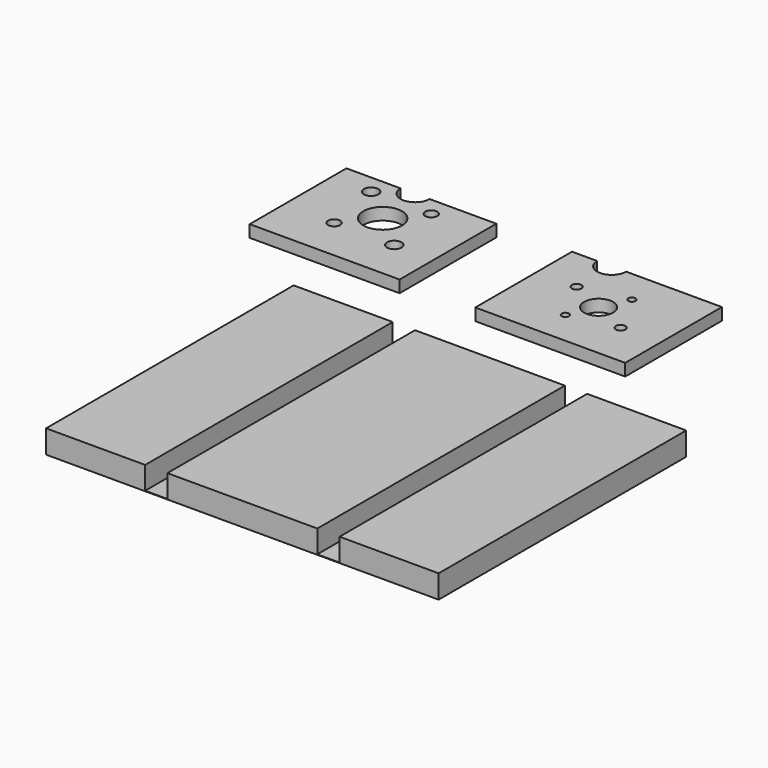
from build123d import *

# Parameters (mm, degrees)
F1_R     = 0.75
F1_R_2   = 1
F1_R_3   = 3
F4_DEPTH = 2.5
F2_R     = 1.25
F2_R_2   = 1.5
F2_R_3   = 4
F3_W     = 4.6
F3_H     = 64
F5_DEPTH = 0.1
F6_DEPTH = 4.7


# Not quite as in the source:
# - ends of sketch curves that miss each other by under 0.0002 mm in the source are joined


with BuildPart() as f4:
    # F1 (on Top) → F4 (new body)
    with BuildSketch(Plane.XY):
        with BuildLine():
            Line((0, 25), (0, 0))
            Line((0, 0), (31, 0))
            Line((31, 0), (31, 25))
            Line((31, 25), (26.3, 25))
            Line((26.3, 25), (11.2, 25))
            ThreePointArc((11.2, 25), (8.2, 22), (5.2, 25))
            Line((5.2, 25), (0, 25))
        make_face()
        with Locations((12.9642904296, 7.0621532778)):
            Circle(F1_R, mode=Mode.SUBTRACT)
        with Locations((22.7504622963, 9.1190539061)):
            Circle(F1_R_2, mode=Mode.SUBTRACT)
        with Locations((8.2495377037, 15.8809460939)):
            Circle(F1_R_2, mode=Mode.SUBTRACT)
        with Locations((15.5, 12.5)):
            Circle(F1_R_3, mode=Mode.SUBTRACT)
        with Locations((18.0357095704, 17.9378467222)):
            Circle(F1_R, mode=Mode.SUBTRACT)
    extrude(amount=F4_DEPTH)


with BuildPart() as f4b:
    # F2 (on Top) → F4, piece 2 (new body)
    with BuildSketch(Plane.XY):
        with BuildLine():
            Line((-46.6549531966, 25), (-46.6549531966, 0))
            Line((-46.6549531966, 0), (-15.6549531966, 0))
            Line((-15.6549531966, 0), (-15.6549531966, 25))
            Line((-15.6549531966, 25), (-20.3549531966, 25))
            Line((-20.3549531966, 25), (-29.4549531966, 25))
            ThreePointArc((-29.4549531966, 25), (-32.4549531966, 22), (-35.4549531966, 25))
            Line((-35.4549531966, 25), (-46.6549531966, 25))
        make_face()
        with Locations((-36.2972540741, 8.871644455)):
            Circle(F2_R, mode=Mode.SUBTRACT)
        with Locations((-23.877530987, 8.893517708)):
            Circle(F2_R_2, mode=Mode.SUBTRACT)
        with Locations((-38.4323754063, 21.106482292)):
            Circle(F2_R_2, mode=Mode.SUBTRACT)
        with Locations((-31.1549531966, 15)):
            Circle(F2_R_3, mode=Mode.SUBTRACT)
        with Locations((-26.0126523192, 21.128355545)):
            Circle(F2_R, mode=Mode.SUBTRACT)
    extrude(amount=F4_DEPTH)


with BuildPart() as f5:
    # F3 (on Top) → F5 (new body)
    with BuildSketch(Plane.XY):
        Polygon((-25.0888298927, -79.5980651379), (-4.6, -79.5980651379), (-4.6, -15.5980651379), (-4.6, -15.5926546171), (-25.1, -15.5926546171), (-25.1, -15.5980651379), align=None)
        Polygon((-4.6, -79.5980651379), (0, -79.5980651379), (0, -15.5980651379), (0, -15.5926546171), (-4.6, -15.5926546171), (-4.6, -15.5980651379), align=None)
        Polygon((0, -15.5980651379), (0, -79.5980651379), (31, -79.5980651379), (31, -15.5980651379), (0, -15.5926546171), align=None)
        with Locations((33.3, -47.5980651379)):
            Rectangle(F3_W, F3_H)
        Polygon((35.6, -15.5980651379), (35.6, -79.5980651379), (56.0888298927, -79.5980651379), (56.1, -15.5980651379), align=None)
    extrude(amount=-F5_DEPTH)

    # F3 (on Top) → F6 (join)
    with BuildSketch(Plane.XY):
        Polygon((-25.0888298927, -79.5980651379), (-4.6, -79.5980651379), (-4.6, -15.5980651379), (-4.6, -15.5926546171), (-25.1, -15.5926546171), (-25.1, -15.5980651379), align=None)
        Polygon((0, -15.5980651379), (0, -79.5980651379), (31, -79.5980651379), (31, -15.5980651379), (0, -15.5926546171), align=None)
        Polygon((35.6, -15.5980651379), (35.6, -79.5980651379), (56.0888298927, -79.5980651379), (56.1, -15.5980651379), align=None)
    extrude(amount=F6_DEPTH)


solid = Compound([f4.part, f4b.part, f5.part])
